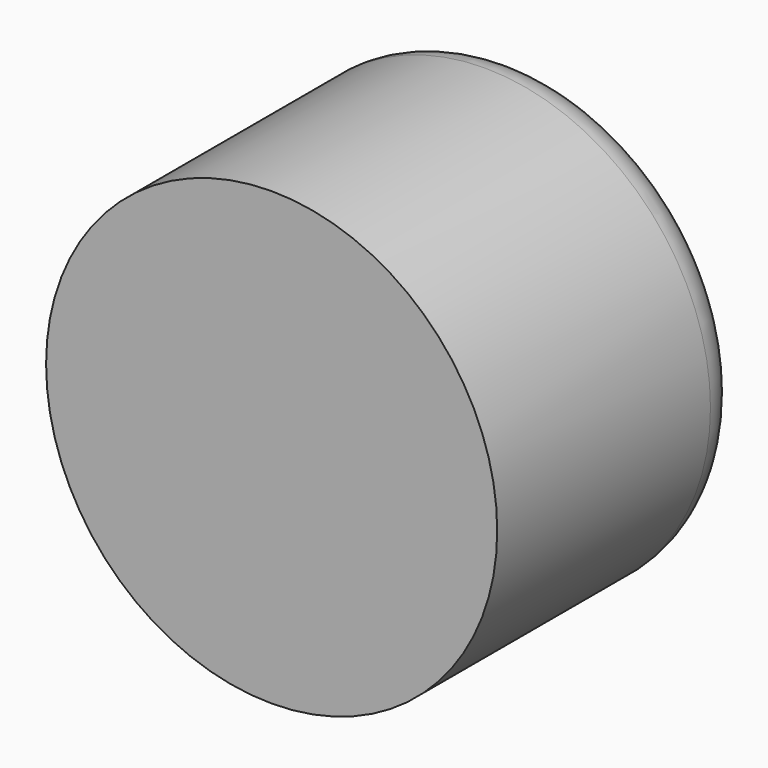
from build123d import *

# Parameters (mm, degrees)
F0_R     = 13.97
F1_DEPTH = 19.05
F2_R     = 2.54


# Not quite as in the source:
# - a feature names something its author has since deleted; it is built from what else it names


with BuildPart() as f1:
    # F0 (on Front) → F1 (new body)
    with BuildSketch(Plane.XZ):
        with Locations((-63.3578656336, 0)):
            Circle(F0_R)
    extrude(amount=-F1_DEPTH)

    # F2
    f2_edges = [f1.edges().sort_by_distance(p)[0] for p in [
        (-77.327866, 19.05, 0),
    ]]
    fillet(f2_edges, radius=F2_R)


with BuildPart() as f1_1:
    # F3: moved
    add(f1.part.moved(Location((65.786, 0, 0))))


solid = f1_1.part
